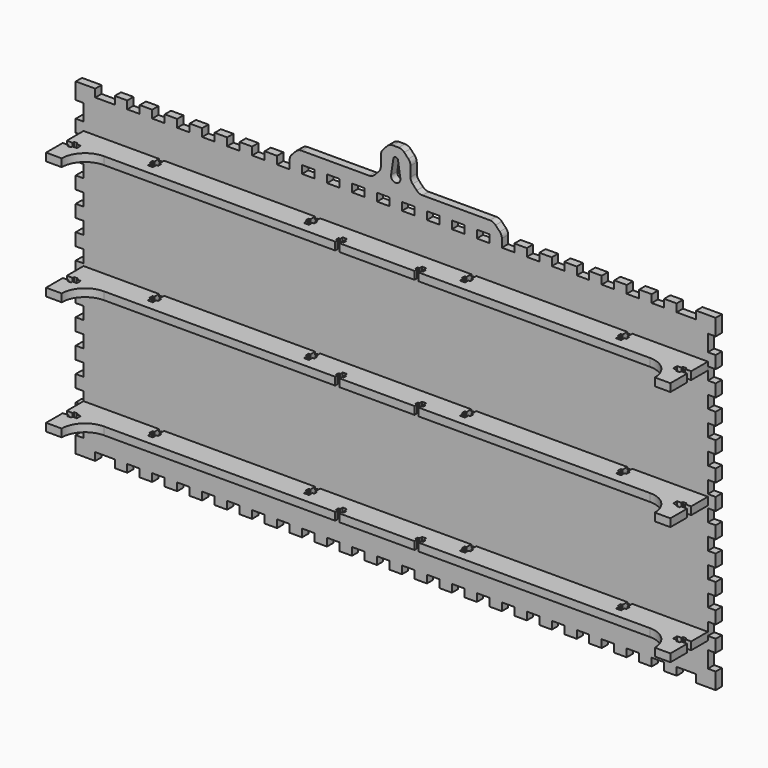
from build123d import *

# Parameters (mm, degrees)
F1_DEPTH = 5
F3_DEPTH = 5
F4_W     = 400.000326
F4_H     = 5
F5_DEPTH = 30
F7_DEPTH = 213.701089
F8_W     = 3.8
F8_H     = 3.2
F8_W_2   = 2.4
F8_W_3   = 2.8
F8_H_2   = 1.15
F8_W_4   = 3.2
F8_H_3   = 2.8
F8_H_4   = 2.4
F8_H_5   = 3.8
F8_W_5   = 1.15
F8_W_6   = 2.7
F8_H_6   = 2
F9_DEPTH = 213.701089
F11_D    = 3.4


with BuildPart() as f1:
    # F0 (on Front) → F1 (new body)
    with BuildSketch(Plane.XZ):
        Polygon((-92.000078, 105.000089), (-100.000085, 105.000089), (-100.000085, 100.000085), (-108.000092, 100.000085), (-108.000092, 105.000089), (-116.000099, 105.000089), (-116.000099, 100.000085), (-124.000105, 100.000085), (-124.000105, 105.000089), (-132.000112, 105.000089), (-132.000112, 100.000085), (-140.000119, 100.000085), (-140.000119, 105.000089), (-148.000126, 105.000089), (-148.000126, 100.000085), (-156.000133, 100.000085), (-156.000133, 105.000089), (-164.000139, 105.000089), (-164.000139, 100.000085), (-172.000146, 100.000085), (-172.000146, 105.000089), (-180.000153, 105.000089), (-180.000153, 100.000085), (-192.500164, 100.000085), (-192.500164, 105.000089), (-205.000174, 105.000089), (-205.000174, 94.50008), (-200.00017, 94.50008), (-200.00017, 84.000071), (-205.000174, 84.000071), (-205.000174, 76.000064), (-200.00017, 76.000064), (-200.00017, 68.000058), (-205.000174, 68.000058), (-205.000174, 60.000051), (-200.00017, 60.000051), (-200.00017, 52.000044), (-205.000174, 52.000044), (-205.000174, 44.000037), (-200.00017, 44.000037), (-200.00017, 36.00003), (-205.000174, 36.00003), (-205.000174, 28.000024), (-200.00017, 28.000024), (-200.00017, 20.000017), (-205.000174, 20.000017), (-205.000174, 12.00001), (-200.00017, 12.00001), (-200.00017, 4.000003), (-205.000174, 4.000003), (-205.000174, -4.000004), (-200.00017, -4.000004), (-200.00017, -12.00001), (-205.000174, -12.00001), (-205.000174, -20.000017), (-200.00017, -20.000017), (-200.00017, -28.000024), (-205.000174, -28.000024), (-205.000174, -36.000031), (-200.00017, -36.000031), (-200.00017, -44.000038), (-205.000174, -44.000038), (-205.000174, -52.000044), (-200.00017, -52.000044), (-200.00017, -60.000051), (-205.000174, -60.000051), (-205.000174, -68.000058), (-200.00017, -68.000058), (-200.00017, -76.000065), (-205.000174, -76.000065), (-205.000174, -84.000072), (-200.00017, -84.000072), (-200.00017, -94.500082), (-205.000174, -94.500082), (-205.000174, -105.000089), (-192.500164, -105.000089), (-192.500164, -100.000085), (-180.000153, -100.000085), (-180.000153, -105.000089), (-172.000146, -105.000089), (-172.000146, -100.000085), (-164.000139, -100.000085), (-164.000139, -105.000089), (-156.000133, -105.000089), (-156.000133, -100.000085), (-148.000126, -100.000085), (-148.000126, -105.000089), (-140.000119, -105.000089), (-140.000119, -100.000085), (-132.000112, -100.000085), (-132.000112, -105.000089), (-124.000105, -105.000089), (-124.000105, -100.000085), (-116.000099, -100.000085), (-116.000099, -105.000089), (-108.000092, -105.000089), (-108.000092, -100.000085), (-100.000085, -100.000085), (-100.000085, -105.000089), (-92.000078, -105.000089), (-92.000078, -100.000085), (-84.000071, -100.000085), (-84.000071, -105.000089), (-76.000065, -105.000089), (-76.000065, -100.000085), (-68.000058, -100.000085), (-68.000058, -105.000089), (-60.000051, -105.000089), (-60.000051, -100.000085), (-52.000044, -100.000085), (-52.000044, -105.000089), (-44.000037, -105.000089), (-44.000037, -100.000085), (-36.000031, -100.000085), (-36.000031, -105.000089), (-28.000024, -105.000089), (-28.000024, -100.000085), (-20.000017, -100.000085), (-20.000017, -105.000089), (-12.00001, -105.000089), (-12.00001, -100.000085), (-4.000003, -100.000085), (-4.000003, -105.000089), (4.000003, -105.000089), (4.000003, -100.000085), (12.00001, -100.000085), (12.00001, -105.000089), (20.000017, -105.000089), (20.000017, -100.000085), (28.000024, -100.000085), (28.000024, -105.000089), (36.000031, -105.000089), (36.000031, -100.000085), (44.000037, -100.000085), (44.000037, -105.000089), (52.000044, -105.000089), (52.000044, -100.000085), (60.000051, -100.000085), (60.000051, -105.000089), (68.000058, -105.000089), (68.000058, -100.000085), (76.000065, -100.000085), (76.000065, -105.000089), (84.000074, -105.000089), (84.000074, -100.000085), (92.000087, -100.000085), (92.000087, -105.000089), (100.000099, -105.000089), (100.000099, -100.000085), (108.000083, -100.000085), (108.000083, -105.000089), (116.000096, -105.000089), (116.000096, -100.000085), (124.000108, -100.000085), (124.000108, -105.000089), (132.000121, -105.000089), (132.000121, -100.000085), (140.000105, -100.000085), (140.000105, -105.000089), (148.000117, -105.000089), (148.000117, -100.000085), (156.00013, -100.000085), (156.00013, -105.000089), (164.000142, -105.000089), (164.000142, -100.000085), (172.000155, -100.000085), (172.000155, -105.000089), (180.000167, -105.000089), (180.000167, -100.000085), (192.500157, -100.000085), (192.500157, -105.000089), (205.000174, -105.000089), (205.000174, -94.500082), (200.000156, -94.500082), (200.000156, -84.000072), (205.000174, -84.000072), (205.000174, -76.000065), (200.000156, -76.000065), (200.000156, -68.000058), (205.000174, -68.000058), (205.000174, -60.000051), (200.000156, -60.000051), (200.000156, -52.000044), (205.000174, -52.000044), (205.000174, -44.000038), (200.000156, -44.000038), (200.000156, -36.000031), (205.000174, -36.000031), (205.000174, -28.000024), (200.000156, -28.000024), (200.000156, -20.000017), (205.000174, -20.000017), (205.000174, -12.00001), (200.000156, -12.00001), (200.000156, -4.000004), (205.000174, -4.000004), (205.000174, 4.000003), (200.000156, 4.000003), (200.000156, 12.00001), (205.000174, 12.00001), (205.000174, 20.000017), (200.000156, 20.000017), (200.000156, 28.000024), (205.000174, 28.000024), (205.000174, 36.00003), (200.000156, 36.00003), (200.000156, 44.000037), (205.000174, 44.000037), (205.000174, 52.000044), (200.000156, 52.000044), (200.000156, 60.000051), (205.000174, 60.000051), (205.000174, 68.000058), (200.000156, 68.000058), (200.000156, 76.000064), (205.000174, 76.000064), (205.000174, 84.000071), (200.000156, 84.000071), (200.000156, 94.50008), (205.000174, 94.50008), (205.000174, 105.000089), (192.500157, 105.000089), (192.500157, 100.000085), (180.000167, 100.000085), (180.000167, 105.000089), (172.000155, 105.000089), (172.000155, 100.000085), (164.000142, 100.000085), (164.000142, 105.000089), (156.00013, 105.000089), (156.00013, 100.000085), (148.000117, 100.000085), (148.000117, 105.000089), (140.000105, 105.000089), (140.000105, 100.000085), (132.000121, 100.000085), (132.000121, 105.000089), (124.000108, 105.000089), (124.000108, 100.000085), (116.000096, 100.000085), (116.000096, 105.000089), (108.000083, 105.000089), (108.000083, 100.000085), (100.000099, 100.000085), (100.000099, 105.000089), (92.000087, 105.000089), (92.000087, 100.000085), (84.000074, 100.000085), (84.000074, 105.000089), (76.000065, 105.000089), (76.000065, 100.000085), (68.000058, 100.000085), (68.000058, 105.000089), (60.000051, 105.000089), (60.000051, 100.000085), (52.000044, 100.000085), (52.000044, 105.000089), (44.000037, 105.000089), (44.000037, 100.000085), (36.000031, 100.000085), (36.000031, 105.000089), (28.000024, 105.000089), (28.000024, 100.000085), (20.000017, 100.000085), (20.000017, 105.000089), (12.00001, 105.000089), (12.00001, 100.000085), (4.000003, 100.000085), (4.000003, 105.000089), (-4.000003, 105.000089), (-4.000003, 100.000085), (-12.00001, 100.000085), (-12.00001, 105.000089), (-20.000017, 105.000089), (-20.000017, 100.000085), (-28.000024, 100.000085), (-28.000024, 105.000089), (-36.000031, 105.000089), (-36.000031, 100.000085), (-44.000037, 100.000085), (-44.000037, 105.000089), (-52.000044, 105.000089), (-52.000044, 100.000085), (-60.000051, 100.000085), (-60.000051, 105.000089), (-68.000058, 105.000089), (-68.000058, 100.000085), (-76.000065, 100.000085), (-76.000065, 105.000089), (-84.000071, 105.000089), (-84.000071, 100.000085), (-92.000078, 100.000085), align=None)
    extrude(amount=F1_DEPTH)

    # F2 (on face) → F3 (join)
    with BuildSketch(Plane.XZ.offset(5)):
        with BuildLine():
            Line((1.8434506048, 135.000089), (0, 135.000089))
            Line((0, 135.000089), (-1.8434506048, 135.000089))
            ThreePointArc((-1.8434506048, 135.000089), (-3.8236635724, 134.5912497033), (-5.4800409891, 133.4315916412))
            Line((-5.4800409891, 133.4315916412), (-8.1269946103, 130.6264397609))
            ThreePointArc((-8.1269946103, 130.6264397609), (-9.1370671103, 129.0411559689), (-9.490404226, 127.1949371197))
            Line((-9.490404226, 127.1949371197), (-9.490404226, 120.8052408803))
            ThreePointArc((-9.490404226, 120.8052408803), (-9.8437413416, 118.9590220311), (-10.8538138417, 117.3737382391))
            Line((-10.8538138417, 117.3737382391), (-13.5007674628, 114.5685863588))
            ThreePointArc((-13.5007674628, 114.5685863588), (-15.1571448796, 113.4089282967), (-17.1373578471, 113.000089))
            Line((-17.1373578471, 113.000089), (-60.3531043788, 113.000089))
            ThreePointArc((-60.3531043788, 113.000089), (-62.3333173464, 112.5912497033), (-63.9896947631, 111.4315916412))
            Line((-63.9896947631, 111.4315916412), (-66.6366483843, 108.6264397609))
            ThreePointArc((-66.6366483843, 108.6264397609), (-67.6467208843, 107.0411559689), (-68.000058, 105.1949371197))
            Line((-68.000058, 105.1949371197), (-68.000058, 105.000089))
            Line((-68.000058, 105.000089), (-60.000051, 105.000089))
            Line((-60.000051, 105.000089), (-52.000044, 105.000089))
            Line((-52.000044, 105.000089), (-44.000037, 105.000089))
            Line((-44.000037, 105.000089), (-36.000031, 105.000089))
            Line((-36.000031, 105.000089), (-28.000024, 105.000089))
            Line((-28.000024, 105.000089), (-20.000017, 105.000089))
            Line((-20.000017, 105.000089), (-12.00001, 105.000089))
            Line((-12.00001, 105.000089), (-4.000003, 105.000089))
            Line((-4.000003, 105.000089), (0, 105.000089))
            Line((0, 105.000089), (4.000003, 105.000089))
            Line((4.000003, 105.000089), (12.00001, 105.000089))
            Line((12.00001, 105.000089), (20.000017, 105.000089))
            Line((20.000017, 105.000089), (28.000024, 105.000089))
            Line((28.000024, 105.000089), (36.000031, 105.000089))
            Line((36.000031, 105.000089), (44.000037, 105.000089))
            Line((44.000037, 105.000089), (52.000044, 105.000089))
            Line((52.000044, 105.000089), (60.000051, 105.000089))
            Line((60.000051, 105.000089), (68.000058, 105.000089))
            Line((68.000058, 105.000089), (68.000058, 105.1949371197))
            ThreePointArc((68.000058, 105.1949371197), (67.6467208843, 107.0411559689), (66.6366483843, 108.6264397609))
            Line((66.6366483843, 108.6264397609), (63.9896947631, 111.4315916412))
            ThreePointArc((63.9896947631, 111.4315916412), (62.3333173464, 112.5912497033), (60.3531043788, 113.000089))
            Line((60.3531043788, 113.000089), (17.1373578471, 113.000089))
            ThreePointArc((17.1373578471, 113.000089), (15.1571448796, 113.4089282967), (13.5007674628, 114.5685863588))
            Line((13.5007674628, 114.5685863588), (10.8538138417, 117.3737382391))
            ThreePointArc((10.8538138417, 117.3737382391), (9.8437413416, 118.9590220311), (9.490404226, 120.8052408803))
            Line((9.490404226, 120.8052408803), (9.490404226, 127.1949371197))
            ThreePointArc((9.490404226, 127.1949371197), (9.1370671103, 129.0411559689), (8.1269946103, 130.6264397609))
            Line((8.1269946103, 130.6264397609), (5.4800409891, 133.4315916412))
            ThreePointArc((5.4800409891, 133.4315916412), (3.8236635724, 134.5912497033), (1.8434506048, 135.000089))
        make_face()
        with BuildLine():
            ThreePointArc((-1.483028995, 127.725089), (0, 129.000089), (1.483028995, 127.725089))
            Line((1.483028995, 127.725089), (2.96605799, 117.950089))
            ThreePointArc((2.96605799, 117.950089), (2.9915024628, 117.7257281256), (3, 117.500089))
            ThreePointArc((3, 117.500089), (-0.2256391256, 114.5085865372), (-2.96605799, 117.950089))
            Line((-2.96605799, 117.950089), (-1.483028995, 127.725089))
        make_face(mode=Mode.SUBTRACT)
    extrude(amount=-F3_DEPTH)

    # F11 (through all)
    with Locations(Plane(origin=(0, 0, 0), x_dir=(-1, 0, 0), z_dir=(0, 1, 0))):
        with Locations((-150, 76.2), (-50, 76.2), (50, 76.2), (150, 76.2), (150, 0), (-50, 0), (50, 0), (-150, -76.2), (150, -76.2), (-50, -76.2), (50, -76.2), (-150, 0)):
            Hole(F11_D / 2)


with BuildPart() as f5:
    # F4 (on face) → F5 (new body)
    with BuildSketch(Plane.XZ.offset(5)):
        with Locations((-7e-06, 0)):
            Rectangle(F4_W, F4_H)
    extrude(amount=F5_DEPTH)


with BuildPart() as f5b:
    # F4 (on face) → F5, piece 2 (new body)
    with BuildSketch(Plane.XZ.offset(5)):
        Polygon((200.000156, 78.7), (-200.00017, 78.7), (-200.00017, 76.000064), (-200.00017, 73.7), (200.000156, 73.7), (200.000156, 76.000064), align=None)
    extrude(amount=F5_DEPTH)


with BuildPart() as f5c:
    # F4 (on face) → F5, piece 3 (new body)
    with BuildSketch(Plane.XZ.offset(5)):
        Polygon((200.000156, -73.7), (-200.00017, -73.7), (-200.00017, -76.000065), (-200.00017, -78.7), (200.000156, -78.7), (200.000156, -76.000065), align=None)
    extrude(amount=F5_DEPTH)


with BuildPart() as f7_tool:
    # F6 (on face) → F7 (new body, through all)
    with BuildSketch(Plane(origin=(0, 0, -78.7), x_dir=(1, 0, 0), z_dir=(0, 0, -1))):
        with BuildLine():
            Line((190.000156, 35), (-190.00017, 35))
            ThreePointArc((-190.00017, 35), (-185.6067717178, 24.3933982822), (-175.00017, 20))
            Line((-175.00017, 20), (175.000156, 20))
            ThreePointArc((175.000156, 20), (185.6067577178, 24.3933982822), (190.000156, 35))
        make_face()
    extrude(amount=-F7_DEPTH)


with BuildPart() as f5_1:
    add(f5.part)

    # F7: cut by f7_tool
    add(f7_tool.part, mode=Mode.SUBTRACT)


with BuildPart() as f5b_1:
    add(f5b.part)

    # F7: cut by f7_tool
    add(f7_tool.part, mode=Mode.SUBTRACT)


with BuildPart() as f5c_1:
    add(f5c.part)

    # F7: cut by f7_tool
    add(f7_tool.part, mode=Mode.SUBTRACT)


with BuildPart() as f9_tool:
    # F8 (on face) → F9 (new body, through all)
    with BuildSketch(Plane(origin=(0, 0, -78.7), x_dir=(1, 0, 0), z_dir=(0, 0, -1))):
        with Locations((-198.10017, 20)):
            Rectangle(F8_W, F8_H)
        with Locations((-195.00017, 20)):
            Rectangle(F8_W_2, F8_H)
        with Locations((-192.40017, 20)):
            Rectangle(F8_W_3, F8_H)
        with Locations((-195.00017, 22.175)):
            Rectangle(F8_W_2, F8_H_2)
        with Locations((-195.00017, 17.825)):
            Rectangle(F8_W_2, F8_H_2)
        with Locations((-150, 12.6)):
            Rectangle(F8_W_4, F8_H_3)
        with Locations((-150, 10)):
            Rectangle(F8_W_4, F8_H_4)
        with Locations((-150, 6.9)):
            Rectangle(F8_W_4, F8_H_5)
        with Locations((-152.175, 10)):
            Rectangle(F8_W_5, F8_H_4)
        with Locations((-147.825, 10)):
            Rectangle(F8_W_5, F8_H_4)
        with Locations((-50, 10)):
            Rectangle(F8_W_4, F8_H_4)
        with Locations((-50, 12.6)):
            Rectangle(F8_W_4, F8_H_3)
        with Locations((-50, 6.9)):
            Rectangle(F8_W_4, F8_H_5)
        with Locations((-47.825, 10)):
            Rectangle(F8_W_5, F8_H_4)
        with Locations((-52.175, 10)):
            Rectangle(F8_W_5, F8_H_4)
        with Locations((-25.4, 19)):
            Rectangle(F8_W_6, F8_H_6)
        with Locations((-27.325, 17)):
            Rectangle(F8_W_5, F8_H_6)
        with Locations((-23.475, 17)):
            Rectangle(F8_W_5, F8_H_6)
        with Locations((-25.4, 15)):
            Rectangle(F8_W_6, F8_H_6)
        with Locations((-25.4, 17)):
            Rectangle(F8_W_6, F8_H_6)
        with Locations((25.4, 19)):
            Rectangle(F8_W_6, F8_H_6)
        with Locations((25.4, 17)):
            Rectangle(F8_W_6, F8_H_6)
        with Locations((23.475, 17)):
            Rectangle(F8_W_5, F8_H_6)
        with Locations((25.4, 15)):
            Rectangle(F8_W_6, F8_H_6)
        with Locations((27.325, 17)):
            Rectangle(F8_W_5, F8_H_6)
        with Locations((50, 12.6)):
            Rectangle(F8_W_4, F8_H_3)
        with Locations((50, 10)):
            Rectangle(F8_W_4, F8_H_4)
        with Locations((50, 6.9)):
            Rectangle(F8_W_4, F8_H_5)
        with Locations((52.175, 10)):
            Rectangle(F8_W_5, F8_H_4)
        with Locations((47.825, 10)):
            Rectangle(F8_W_5, F8_H_4)
        with Locations((150, 10)):
            Rectangle(F8_W_4, F8_H_4)
        with Locations((150, 12.6)):
            Rectangle(F8_W_4, F8_H_3)
        with Locations((150, 6.9)):
            Rectangle(F8_W_4, F8_H_5)
        with Locations((147.825, 10)):
            Rectangle(F8_W_5, F8_H_4)
        with Locations((152.175, 10)):
            Rectangle(F8_W_5, F8_H_4)
        with Locations((198.10017, 20)):
            Rectangle(F8_W, F8_H)
        with Locations((195.00017, 20)):
            Rectangle(F8_W_2, F8_H)
        with Locations((195.00017, 22.175)):
            Rectangle(F8_W_2, F8_H_2)
        with Locations((195.00017, 17.825)):
            Rectangle(F8_W_2, F8_H_2)
        with Locations((192.40017, 20)):
            Rectangle(F8_W_3, F8_H)
    extrude(amount=-F9_DEPTH)


with BuildPart() as f5_2:
    add(f5_1.part)

    # F9: cut by f9_tool
    add(f9_tool.part, mode=Mode.SUBTRACT)


with BuildPart() as f5b_2:
    add(f5b_1.part)

    # F9: cut by f9_tool
    add(f9_tool.part, mode=Mode.SUBTRACT)


with BuildPart() as f5c_2:
    add(f5c_1.part)

    # F9: cut by f9_tool
    add(f9_tool.part, mode=Mode.SUBTRACT)


solid = Compound([f1.part, f5_2.part, f5b_2.part, f5c_2.part])
